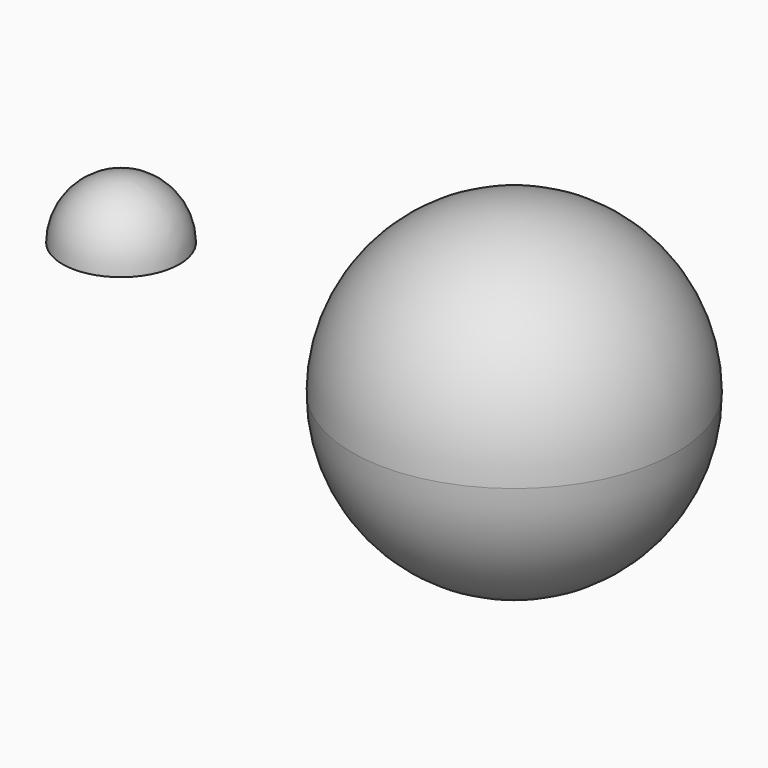
from build123d import *


# Not quite as in the source:
# - ends of sketch curves that miss each other by under 0.0002 mm in the source are joined


with BuildPart() as f1:
    # F0 (on Front) → F1 (revolve)
    with BuildSketch(Plane.XZ):
        with BuildLine():
            ThreePointArc((-10.3562049295, -7.0185781017), (8.7236423428, 0.8845534065), (16.626773851, 19.9644006789))
            ThreePointArc((16.626773851, 19.9644006789), (8.7236423428, 39.0442479512), (-10.3562049295, 46.9473794594))
            Line((-10.3562049295, 46.9473794594), (-10.3562049295, -7.0185781017))
        make_face()
    revolve(axis=Axis((-10.3562049295, 0, 19.9644006789), (0, 0, -1)))


with BuildPart() as f3:
    # F2 (on Front) → F3 (revolve)
    with BuildSketch(Plane.XZ):
        with BuildLine():
            Line((-75.7629424334, 20.6659585238), (-66.0263107651, 20.6659585238))
            ThreePointArc((-66.0263107651, 20.6659585238), (-68.8781041548, 27.5507968023), (-75.7629424334, 30.402590192))
            Line((-75.7629424334, 30.402590192), (-75.7629424334, 20.6659585238))
        make_face()
    revolve(axis=Axis((-75.7629424334, 0, 25.5342743579), (0, 0, 1)))


solid = Compound([f1.part, f3.part])
